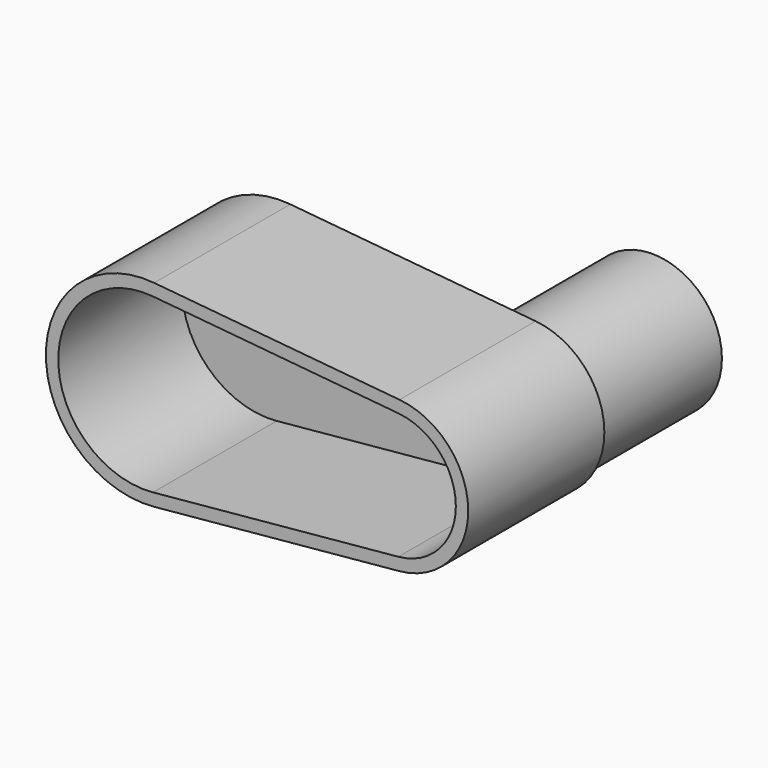
from build123d import *

# Parameters (mm, degrees)
F0_R     = 20
F1_DEPTH = 5
F2_DEPTH = 50
F4_DEPTH = 5
F5_DEPTH = 50


with BuildPart() as f1:
    # F0 (on Front) → F1 (new body)
    with BuildSketch(Plane.XZ):
        with BuildLine():
            ThreePointArc((-10, 0), (-17.8147008134, 20.1943680268), (-37.1875, 29.8678731039))
            ThreePointArc((-37.1875, 29.8678731039), (-70, 0), (-37.1875, -29.8678731039))
            ThreePointArc((-37.1875, -29.8678731039), (-17.8147008134, -20.1943680268), (-10, 0))
        make_face()
        with BuildLine():
            ThreePointArc((42.109375, -22.4009048279), (17.5, 0), (42.109375, 22.4009048279))
            Line((42.109375, 22.4009048279), (-37.1875, 29.8678731039))
            ThreePointArc((-37.1875, 29.8678731039), (-17.8147008134, 20.1943680268), (-10, 0))
            ThreePointArc((-10, 0), (-17.8147008134, -20.1943680268), (-37.1875, -29.8678731039))
            Line((-37.1875, -29.8678731039), (42.109375, -22.4009048279))
        make_face()
        with BuildLine():
            ThreePointArc((42.109375, -22.4009048279), (56.63897439, -15.1457760201), (62.5, 0))
            ThreePointArc((62.5, 0), (56.63897439, 15.1457760201), (42.109375, 22.4009048279))
            ThreePointArc((42.109375, 22.4009048279), (17.5, 0), (42.109375, -22.4009048279))
        make_face()
        with Locations((40, 0)):
            Circle(F0_R, mode=Mode.SUBTRACT)
    extrude(amount=F1_DEPTH)

    # F0 (on Front) → F2 (join)
    with BuildSketch(Plane.XZ):
        with BuildLine():
            ThreePointArc((42.109375, -22.4009048279), (56.63897439, -15.1457760201), (62.5, 0))
            ThreePointArc((62.5, 0), (56.63897439, 15.1457760201), (42.109375, 22.4009048279))
            ThreePointArc((42.109375, 22.4009048279), (17.5, 0), (42.109375, -22.4009048279))
        make_face()
        with Locations((40, 0)):
            Circle(F0_R, mode=Mode.SUBTRACT)
    extrude(amount=-F2_DEPTH)


with BuildPart() as f4:
    # F3 (on face) → F4 (new body)
    with BuildSketch(Plane.XZ.offset(5)):
        with BuildLine():
            ThreePointArc((-37, 31.8590646441), (-72, 0), (-37, -31.8590646441))
            Line((-37, -31.8590646441), (42.296875, -24.3920963682))
            ThreePointArc((42.296875, -24.3920963682), (64.5, 0), (42.296875, 24.3920963682))
            Line((42.296875, 24.3920963682), (-37, 31.8590646441))
        make_face()
        with BuildLine():
            ThreePointArc((-37.1875, -29.8678731039), (-70, 0), (-37.1875, 29.8678731039))
            Line((-37.1875, 29.8678731039), (42.109375, 22.4009048279))
            ThreePointArc((42.109375, 22.4009048279), (62.5, 0), (42.109375, -22.4009048279))
            Line((42.109375, -22.4009048279), (-37.1875, -29.8678731039))
        make_face(mode=Mode.SUBTRACT)
    extrude(amount=-F4_DEPTH)

    # F3 (on face) → F5 (join)
    with BuildSketch(Plane.XZ.offset(5)):
        with BuildLine():
            ThreePointArc((-37, 31.8590646441), (-72, 0), (-37, -31.8590646441))
            Line((-37, -31.8590646441), (42.296875, -24.3920963682))
            ThreePointArc((42.296875, -24.3920963682), (64.5, 0), (42.296875, 24.3920963682))
            Line((42.296875, 24.3920963682), (-37, 31.8590646441))
        make_face()
        with BuildLine():
            ThreePointArc((-37.1875, -29.8678731039), (-70, 0), (-37.1875, 29.8678731039))
            Line((-37.1875, 29.8678731039), (42.109375, 22.4009048279))
            ThreePointArc((42.109375, 22.4009048279), (62.5, 0), (42.109375, -22.4009048279))
            Line((42.109375, -22.4009048279), (-37.1875, -29.8678731039))
        make_face(mode=Mode.SUBTRACT)
        with BuildLine():
            Line((42.109375, 22.4009048279), (-37.1875, 29.8678731039))
            ThreePointArc((-37.1875, 29.8678731039), (-70, 0), (-37.1875, -29.8678731039))
            Line((-37.1875, -29.8678731039), (42.109375, -22.4009048279))
            ThreePointArc((42.109375, -22.4009048279), (62.5, 0), (42.109375, 22.4009048279))
        make_face()
        with BuildLine():
            ThreePointArc((-37.375, -27.8766815636), (-68, 0), (-37.375, 27.8766815636))
            Line((-37.375, 27.8766815636), (41.921875, 20.4097132877))
            ThreePointArc((41.921875, 20.4097132877), (60.5, 0), (41.921875, -20.4097132877))
            Line((41.921875, -20.4097132877), (-37.375, -27.8766815636))
        make_face(mode=Mode.SUBTRACT)
    extrude(amount=F5_DEPTH)


solid = Compound([f1.part, f4.part])
